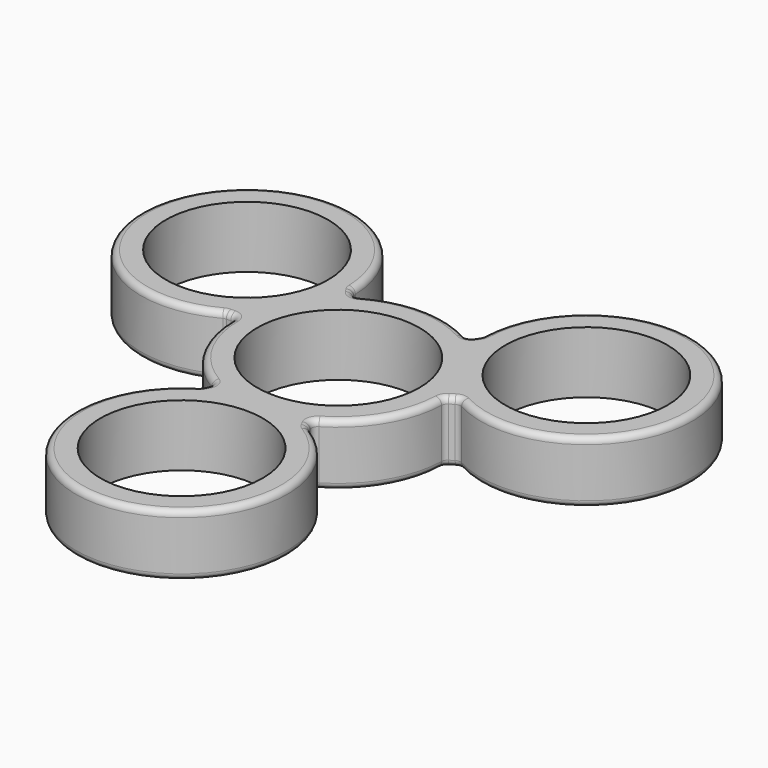
from build123d import *

# Parameters (mm, degrees)
F1_R     = 6.575
F2_DEPTH = 5
F3_R     = 0.5


with BuildPart() as f2:
    # F1 (on Top) → F2 (new body)
    with BuildSketch(Plane.XY):
        with BuildLine():
            Line((-4.6323397162, 7.2160968503), (-5.1725542604, 8.0576241798))
            ThreePointArc((-5.1725542604, 8.0576241798), (-21.1732346231, 12.2235279993), (-9.5631071668, 0.4514650047))
            Line((-9.5631071668, 0.4514650047), (-8.5631071668, 0.4514650047))
            ThreePointArc((-8.5631071668, 0.4514650047), (-7.4141766645, 4.3082025704), (-4.6323397162, 7.2160968503))
        make_face()
        with Locations((-13.7467010425, 7.9366615474)):
            Circle(F1_R, mode=Mode.SUBTRACT)
        with BuildLine():
            Line((5.1725542604, 8.0576241798), (4.6323397162, 7.2160968503))
            ThreePointArc((4.6323397162, 7.2160968503), (7.5250560817, 4.111466401), (8.575, 0))
            Line((8.575, 0), (9.4215003257, 0.5323882029))
            ThreePointArc((9.4215003257, 0.5323882029), (21.2136673342, 12.1527070165), (5.1725542604, 8.0576241798))
        make_face()
        with Locations((13.7467010425, 7.9366615474)):
            Circle(F1_R, mode=Mode.SUBTRACT)
        with BuildLine():
            ThreePointArc((3.9331533305, -7.6197722984), (0, -8.575), (-3.9331533305, -7.6197722984))
            Line((-3.9331533305, -7.6197722984), (-4.3918301037, -8.5083754819))
            ThreePointArc((-4.3918301037, -8.5083754819), (0, -24.4483230947), (4.3918301037, -8.5083754819))
            Line((4.3918301037, -8.5083754819), (3.9331533305, -7.6197722984))
        make_face()
        with Locations((0, -15.8733230947)):
            Circle(F1_R, mode=Mode.SUBTRACT)
        with BuildLine():
            ThreePointArc((4.6323397162, 7.2160968503), (0, 8.575), (-4.6323397162, 7.2160968503))
            ThreePointArc((-4.6323397162, 7.2160968503), (-7.4141766645, 4.3082025704), (-8.5631071668, 0.4514650047))
            ThreePointArc((-8.5631071668, 0.4514650047), (-7.4381012029, -4.2667640544), (-3.9331533305, -7.6197722984))
            ThreePointArc((-3.9331533305, -7.6197722984), (0, -8.575), (3.9331533305, -7.6197722984))
            ThreePointArc((3.9331533305, -7.6197722984), (7.323162391, -4.4611565312), (8.575, 0))
            ThreePointArc((8.575, 0), (7.5250560817, 4.111466401), (4.6323397162, 7.2160968503))
        make_face()
        Circle(F1_R, mode=Mode.SUBTRACT)
    extrude(amount=F2_DEPTH)

    # F3
    f3_edges = [f2.edges().sort_by_distance(p)[0] for p in [
        (-5.172554, 8.057624, 2.5),
        (-9.563107, 0.451465, 2.5),
        (-21.173235, 12.223528, 0),
        (-21.173235, 12.223528, 5),
        (-8.563107, 0.451465, 2.5),
        (-3.933153, -7.619772, 2.5),
        (-7.438101, -4.266764, 0),
        (-7.438101, -4.266764, 5),
        (-4.39183, -8.508375, 2.5),
        (4.39183, -8.508375, 2.5),
        (0, -24.448323, 0),
        (0, -24.448323, 5),
        (-9.063107, 0.451465, 0),
        (-9.063107, 0.451465, 5),
        (-4.162492, -8.064074, 0),
        (-4.162492, -8.064074, 5),
        (3.933153, -7.619772, 2.5),
        (4.162492, -8.064074, 0),
        (4.162492, -8.064074, 5),
        (8.575, 0, 2.5),
        (7.323162, -4.461157, 0),
        (7.323162, -4.461157, 5),
        (9.4215, 0.532388, 2.5),
        (5.172554, 8.057624, 2.5),
        (21.213667, 12.152707, 0),
        (21.213667, 12.152707, 5),
        (4.63234, 7.216097, 2.5),
        (4.902447, 7.636861, 0),
        (4.902447, 7.636861, 5),
        (-4.63234, 7.216097, 2.5),
        (0, 8.575, 0),
        (0, 8.575, 5),
        (-4.902447, 7.636861, 0),
        (-4.902447, 7.636861, 5),
        (8.99825, 0.266194, 0),
        (8.99825, 0.266194, 5),
    ]]
    fillet(f3_edges, radius=F3_R)


solid = f2.part
